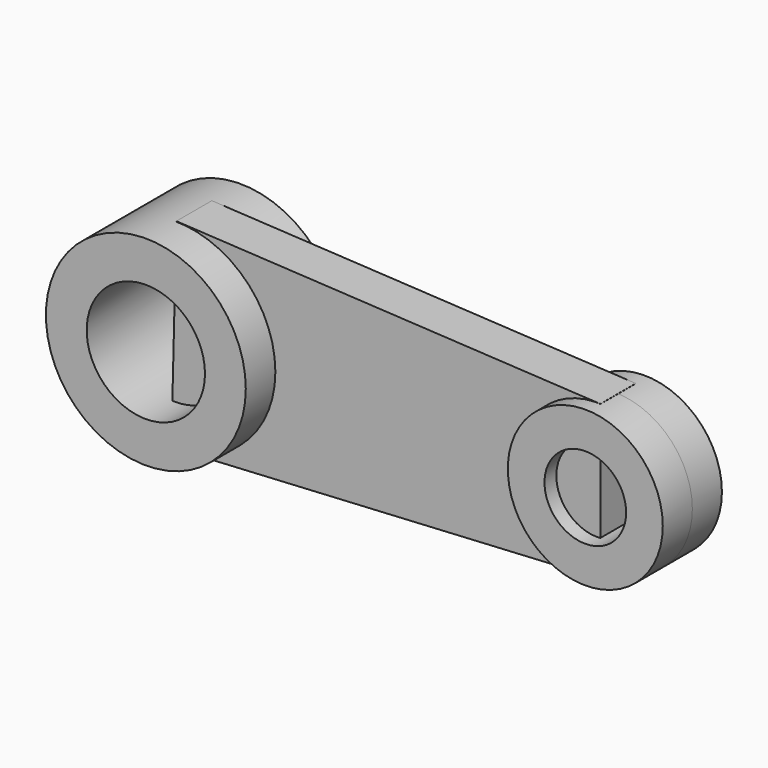
from build123d import *

# Parameters (mm, degrees)
F0_R          = 42.926
F2_DEPTH      = 25.4
F2_DEPTH_BACK = 25.4
F1_R          = 33.274
F3_DEPTH      = 15.875
F3_DEPTH_BACK = 15.875
F5_DEPTH      = 9.525
F5_DEPTH_BACK = 9.525
F6_R          = 25.4
F7_DEPTH      = 132.39676
F8_R          = 17.526
F9_DEPTH      = 95.20603


with BuildPart() as f2:
    # F0 (on Front) → F2 (new body, two sides)
    with BuildSketch(Plane.XZ) as f2_sk:
        with Locations((-91.0871326923, 0)):
            Circle(F0_R)
    extrude(amount=F2_DEPTH)
    extrude(f2_sk.sketch, amount=-F2_DEPTH_BACK)

    # F6 (on face) → F7 (cut)
    with BuildSketch(Plane.XZ.offset(25.4)):
        with Locations((-91.0871326923, 0)):
            Circle(F6_R)
    extrude(amount=-F7_DEPTH, mode=Mode.SUBTRACT)


with BuildPart() as f3:
    # F1 (on Front) → F3 (new body, two sides)
    with BuildSketch(Plane.XZ) as f3_sk:
        with Locations((90.0334119797, 0)):
            Circle(F1_R)
    extrude(amount=-F3_DEPTH)
    extrude(f3_sk.sketch, amount=F3_DEPTH_BACK)

    # F8 (on face) → F9 (cut)
    with BuildSketch(Plane.XZ.offset(15.875)):
        with Locations((90.0334119797, 0)):
            Circle(F8_R)
    extrude(amount=-F9_DEPTH, mode=Mode.SUBTRACT)


with BuildPart() as f5:
    # F4 (on Front) → F5 (new body, two sides)
    with BuildSketch(Plane.XZ) as f5_sk:
        Polygon((91.4073139429, 33.2323312759), (-90.6749367714, 43.1247465312), (-92.8388983011, -43.1247465312), (91.4073139429, -32.9231917858), align=None)
    extrude(amount=F5_DEPTH)
    extrude(f5_sk.sketch, amount=-F5_DEPTH_BACK)


solid = Compound([f2.part, f3.part, f5.part])
